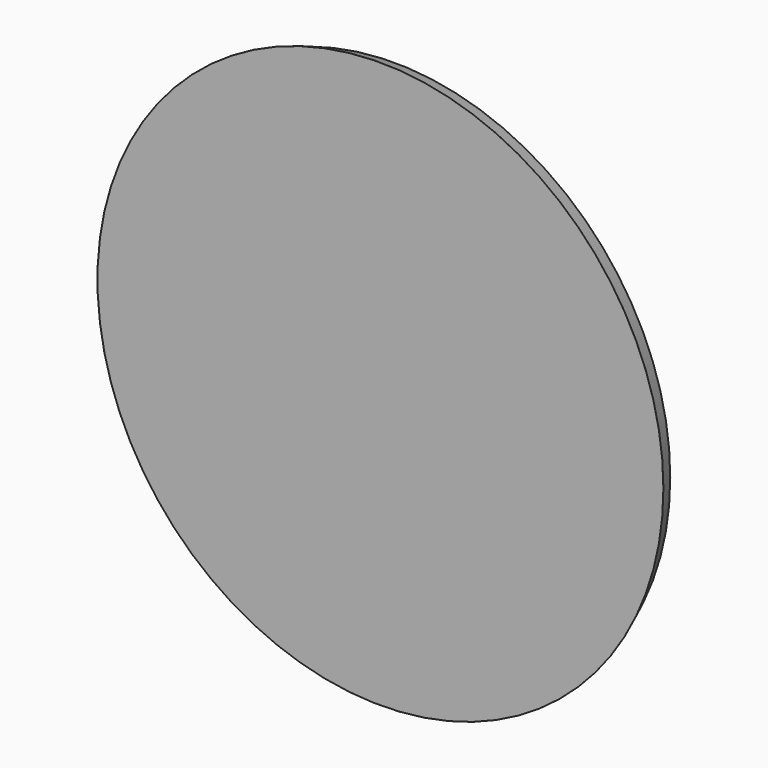
from build123d import *

# Parameters (mm, degrees)
F0_R     = 62.3719654877
F1_DEPTH = 3.5956986248
F3_SIZE  = 5.08


# Not quite as in the source:
# - a fillet or chamfer that OpenCascade refuses, or shapes differently, is made with other operations: its cross-section is extruded or revolved along the edge and cut away or added


with BuildPart() as f1:
    # F0 (on Front) → F1 (new body)
    with BuildSketch(Plane.XZ):
        with Locations((-8.0392340643, 1.049432549)):
            Circle(F0_R)
    extrude(amount=-F1_DEPTH)

    # F2: chamfer of 5.08 on 1 edges, made by hand

    # F2_s1 → F2_t2 (revolve, cut)
    with BuildSketch(Plane.XY.offset(1.049432549)):
        Polygon((54.3327314234, 5.08), (49.2527314234, 0), (54.3327314234, 0), align=None)
    revolve(axis=Axis((-8.0392340643, 0, 1.049432549), (0, -1, 0)), mode=Mode.SUBTRACT)

    # F3
    f3_edges = [f1.edges().sort_by_distance(p)[0] for p in [
        (-68.926898, 3.595699, 1.049433),
    ]]
    chamfer(f3_edges, length=F3_SIZE)


solid = f1.part
